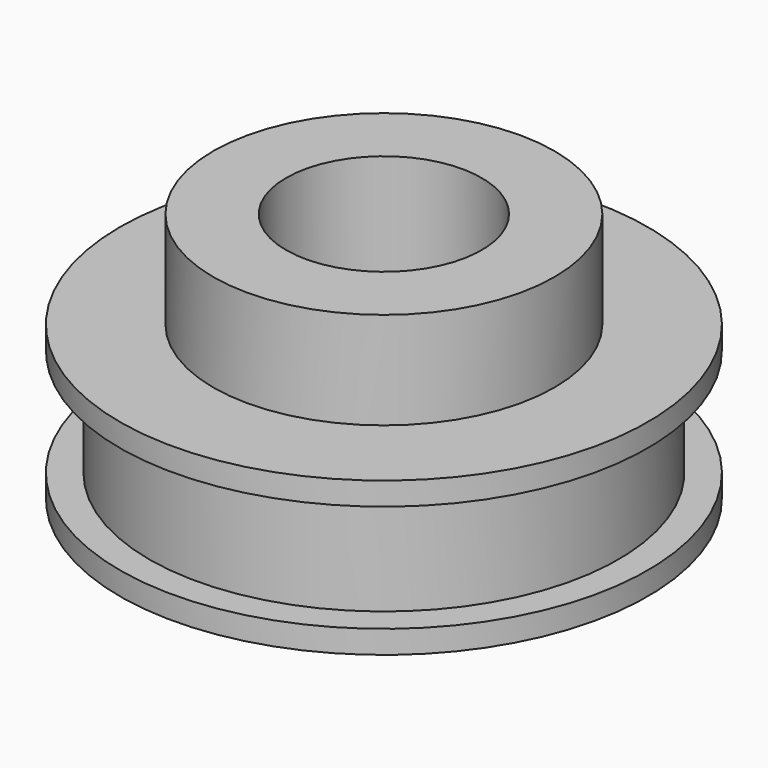
from build123d import *

# Parameters (mm, degrees)
F0_W = 7.45
F0_H = 9.95


# Not quite as in the source:
# - a feature names something its author has since deleted; it is built from what else it names


with BuildPart() as f1:
    # F0 (on Front) → F1 (revolve)
    with BuildSketch(Plane.XZ):
        Polygon((0, 2.35), (0, 0), (17, 0), (17, 15.7), (9.55, 15.7), (0, 15.7), (0, 13.35), (3, 13.35), (3, 2.35), align=None)
        with Locations((13.275, 20.675)):
            Rectangle(F0_W, F0_H)
    revolve(axis=Axis((27, 0, 7.85), (0, 0, 1)))


solid = f1.part
